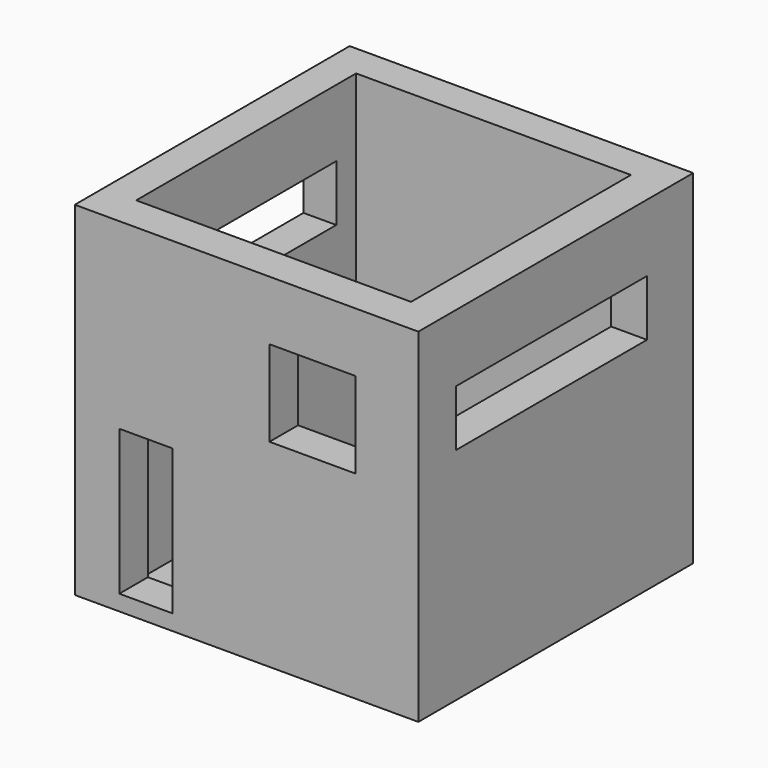
from build123d import *

# Parameters (mm, degrees)
F0_W     = 50.8
F0_H     = 50.8
F1_DEPTH = 50.8
F2_W     = 40.64
F2_H     = 40.64
F3_DEPTH = 49.53
F4_W     = 7.850907743
F4_H     = 21.4745448902
F5_DEPTH = 25.4
F6_W     = 12.7
F6_H     = 12.7
F7_DEPTH = 7.62
F8_W     = 35.329092294
F8_H     = 8.312728256
F9_DEPTH = 50.8


with BuildPart() as f1:
    # F0 (on Top) → F1 (new body)
    with BuildSketch(Plane.XY):
        with Locations((2.078182064, 0.7973827244)):
            Rectangle(F0_W, F0_H)
    extrude(amount=F1_DEPTH)

    # F2 (on face) → F3 (cut)
    with BuildSketch(Plane.XY.offset(50.8)):
        with Locations((1.8472736701, 1.0047121724)):
            Rectangle(F2_W, F2_H)
    extrude(amount=-F3_DEPTH, mode=Mode.SUBTRACT)

    # F4 (on face) → F5 (cut)
    with BuildSketch(Plane.XZ.offset(24.6026172756)):
        with Locations((-12.8154549748, 13.0454613827)):
            Rectangle(F4_W, F4_H)
    extrude(amount=-F5_DEPTH, mode=Mode.SUBTRACT)

    # F6 (on face) → F7 (cut)
    with BuildSketch(Plane.XZ.offset(24.6026172756)):
        with Locations((11.8126636371, 35.6554915783)):
            Rectangle(F6_W, F6_H)
    extrude(amount=-F7_DEPTH, mode=Mode.SUBTRACT)

    # F8 (on face) → F9 (cut)
    with BuildSketch(Plane(origin=(-23.321817936, 0, 0), x_dir=(0, -1, 0), z_dir=(-1, 0, 0))):
        with Locations((0, 36.7136429995)):
            Rectangle(F8_W, F8_H)
    extrude(amount=-F9_DEPTH, mode=Mode.SUBTRACT)


solid = f1.part
